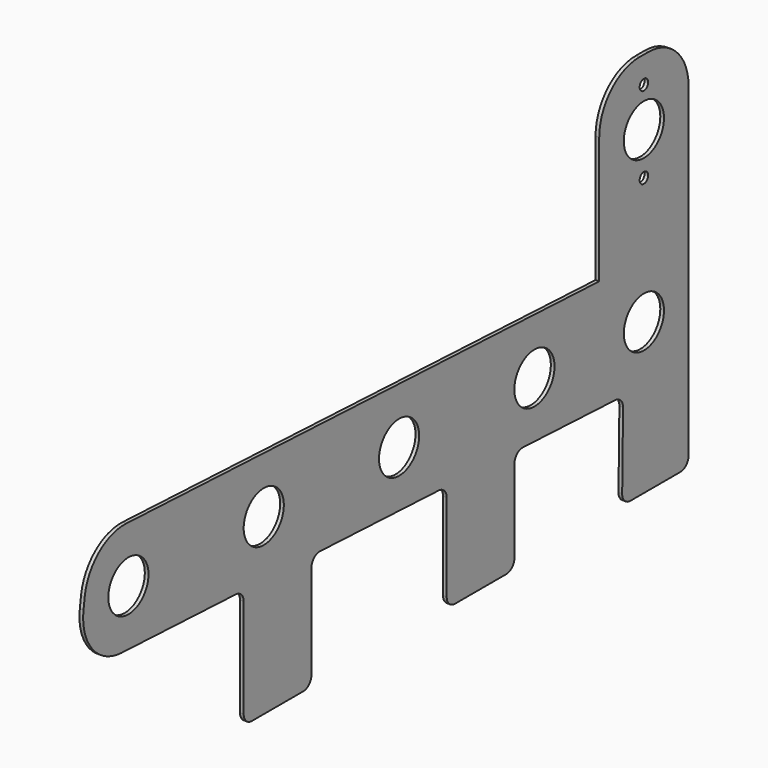
from build123d import *

# Parameters (mm, degrees)
F0_R     = 15.5702
F0_R_2   = 3.302
F1_DEPTH = 2.286


# Not quite as in the source:
# - a feature names something its author has since deleted; it is built from what else it names


with BuildPart() as f1:
    # F0 (on Right) → F1 (new body)
    with BuildSketch(Plane.YZ):
        with BuildLine():
            Line((-45.1142073236, -26.818738899), (-411.6793204181, -9.9719436831))
            ThreePointArc((-411.6793204181, -9.9719436831), (-433.0208080629, -17.1370033148), (-443.9559804746, -36.8148888401))
            Line((-443.9559804746, -36.8148888401), (-444.9130844184, -43.7378478567))
            ThreePointArc((-444.9130844184, -43.7378478567), (-438.0085876413, -67.9142971029), (-415.4957405146, -79.1100323691))
            Line((-415.4957405146, -79.1100323691), (-326.7930180723, -83.186679455))
            ThreePointArc((-326.7930180723, -83.186679455), (-322.4925045261, -85.1441378233), (-320.7345470438, -89.5299838666))
            Line((-320.7345470438, -89.5299838666), (-320.7345470438, -151.0368096017))
            ThreePointArc((-320.7345470438, -151.0368096017), (-318.8746751043, -155.5269376622), (-314.3845470438, -157.3868096017))
            Line((-314.3845470438, -157.3868096017), (-274.5700470438, -157.3868096017))
            ThreePointArc((-274.5700470438, -157.3868096017), (-270.0799189833, -155.5269376622), (-268.2200470438, -151.0368096017))
            Line((-268.2200470438, -151.0368096017), (-268.2200470438, -92.5271466826))
            ThreePointArc((-268.2200470438, -92.5271466826), (-266.2558930871, -87.9351041649), (-261.5785180723, -86.183842271))
            Line((-261.5785180723, -86.183842271), (-169.4194716536, -90.4193369398))
            ThreePointArc((-169.4194716536, -90.4193369398), (-165.1189581074, -92.3767953082), (-163.3610006251, -96.7626413515))
            Line((-163.3610006251, -96.7626413515), (-163.3610006251, -151.0368096017))
            ThreePointArc((-163.3610006251, -151.0368096017), (-161.5011286857, -155.5269376622), (-157.0110006251, -157.3868096017))
            Line((-157.0110006251, -157.3868096017), (-117.1965006251, -157.3868096017))
            ThreePointArc((-117.1965006251, -157.3868096017), (-112.7063725646, -155.5269376622), (-110.8465006251, -151.0368096017))
            Line((-110.8465006251, -151.0368096017), (-110.8465006251, -99.7598041674))
            ThreePointArc((-110.8465006251, -99.7598041674), (-108.8823466684, -95.1677616497), (-104.2049716536, -93.4164997558))
            Line((-104.2049716536, -93.4164997558), (-32.7059788978, -96.7024886458))
            ThreePointArc((-32.7059788978, -96.7024886458), (-28.3737210787, -98.6934263777), (-26.6481782752, -103.1380627967))
            Line((-26.6481782752, -103.1380627967), (-27.3295071805, -150.0221421965))
            ThreePointArc((-27.3295071805, -150.0221421965), (-25.5028102734, -154.5717983424), (-20.9801775863, -156.4644119358))
            Line((-20.9801775863, -156.4644119358), (17.7761926764, -156.4644119358))
            ThreePointArc((17.7761926764, -156.4644119358), (22.266320737, -154.6045399963), (24.1261926764, -150.1144119358))
            Line((24.1261926764, -150.1144119358), (24.1261926764, -99.3144119358))
            Line((24.1261926764, -99.3144119358), (24.1261926764, -36.0657921419))
            ThreePointArc((24.1261926764, -36.0657921419), (22.3682351942, -31.6799460986), (18.0677216479, -29.7224877302))
            Line((18.0677216479, -29.7224877302), (-45.1142073236, -26.818738899))
        make_face()
        with Locations((-410.0968120394, -44.7014163277)):
            Circle(F0_R, mode=Mode.SUBTRACT)
        with Locations((-305.1785570708, -49.5233055166)):
            Circle(F0_R, mode=Mode.SUBTRACT)
        with Locations((-200.2603021023, -54.3451947055)):
            Circle(F0_R, mode=Mode.SUBTRACT)
        with Locations((-95.3420471337, -59.1670838944)):
            Circle(F0_R, mode=Mode.SUBTRACT)
        with Locations((-10.4940073236, -63.0665754174)):
            Circle(F0_R, mode=Mode.SUBTRACT)
        with BuildLine():
            Line((-45.1142073236, 51.7922245826), (-45.1142073236, -26.818738899))
            Line((-45.1142073236, -26.818738899), (18.0677216479, -29.7224877302))
            Line((18.0677216479, -29.7224877302), (24.1261926764, -30.000926177))
            Line((24.1261926764, -30.000926177), (24.1261926764, 51.7922245826))
            ThreePointArc((24.1261926764, 51.7922245826), (15.0053806853, 73.8118125915), (-7.0142073236, 82.9326245826))
            Line((-7.0142073236, 82.9326245826), (-13.9738073236, 82.9326245826))
            ThreePointArc((-13.9738073236, 82.9326245826), (-35.9933953324, 73.8118125915), (-45.1142073236, 51.7922245826))
        make_face()
        with Locations((-10.4940073236, 15.6400269167)):
            Circle(F0_R_2, mode=Mode.SUBTRACT)
        with Locations((-10.4940073236, 41.9624245826)):
            Circle(F0_R, mode=Mode.SUBTRACT)
        with Locations((-10.4940073236, 66.4400269167)):
            Circle(F0_R_2, mode=Mode.SUBTRACT)
        with BuildLine():
            Line((24.1261926764, -30.000926177), (18.0677216479, -29.7224877302))
            ThreePointArc((18.0677216479, -29.7224877302), (22.3682351942, -31.6799460986), (24.1261926764, -36.0657921419))
            Line((24.1261926764, -36.0657921419), (24.1261926764, -30.000926177))
        make_face()
    extrude(amount=F1_DEPTH)


solid = f1.part
